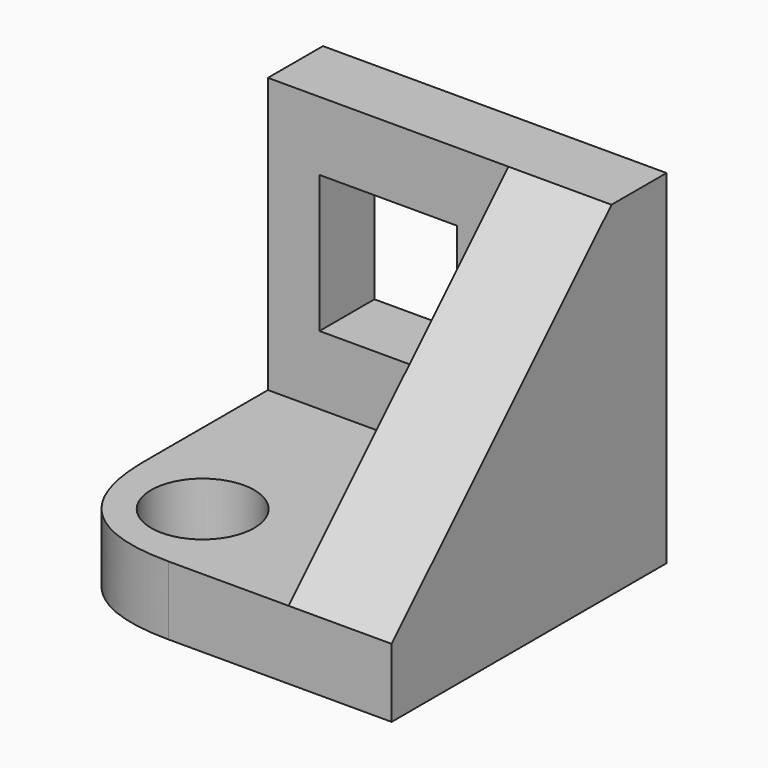
from build123d import *

# Parameters (mm, degrees)
F0_W        = 100
F0_H        = 100
F1_DEPTH    = 20
F2_W        = 100
F2_H        = 20
F3_DEPTH    = 80
F4_R        = 15
F5_DEPTH    = 20
F6_T1_DEPTH = 195
F7_W        = 30
F7_H        = 80
F8_DEPTH    = 80
F9_SIZE     = 80
F10_W       = 40
F10_H       = 40
F11_DEPTH   = 20


# Not quite as in the source:
# - a fillet or chamfer that OpenCascade refuses, or shapes differently, is made with other operations: its cross-section is extruded or revolved along the edge and cut away or added


with BuildPart() as f1:
    # F0 (on Top) → F1 (new body)
    with BuildSketch(Plane.XY):
        Rectangle(F0_W, F0_H)
    extrude(amount=F1_DEPTH)

    # F2 (on face) → F3 (join)
    with BuildSketch(Plane.XY.offset(20)):
        with Locations((0, 40)):
            Rectangle(F2_W, F2_H)
    extrude(amount=F3_DEPTH)

    # F4 (on face) → F5 (cut)
    with BuildSketch(Plane.XY.offset(20)):
        with Locations((-25, -25)):
            Circle(F4_R)
    extrude(amount=-F5_DEPTH, mode=Mode.SUBTRACT)

    # F6: fillet of radius 35 on 1 edges, made by hand

    # F6_s2 → F6_t1 (cut)
    with BuildSketch(Plane.XY.offset(-87.5)):
        with BuildLine():
            add(Edge.make_bspline(
                [(-50, -15), (-50, -50), (-15, -50)],
                knots=[0, 0, 0, 1, 1, 1], degree=2, weights=[1, 1, 1]))
            Line((-15, -50), (-50, -50))
            Line((-50, -50), (-50, -15))
        make_face()
    extrude(amount=F6_T1_DEPTH, mode=Mode.SUBTRACT)

    # F7 (on face) → F8 (join)
    with BuildSketch(Plane.XY.offset(20)):
        with Locations((35, -10)):
            Rectangle(F7_W, F7_H)
    extrude(amount=F8_DEPTH)

    # F9
    f9_edges = [f1.edges().sort_by_distance(p)[0] for p in [
        (35, -50, 100),
    ]]
    chamfer(f9_edges, length=F9_SIZE)

    # F10 (on face) → F11 (cut)
    with BuildSketch(Plane.XZ.offset(-30)):
        with Locations((-15, 60)):
            Rectangle(F10_W, F10_H)
    extrude(amount=-F11_DEPTH, mode=Mode.SUBTRACT)


solid = f1.part
